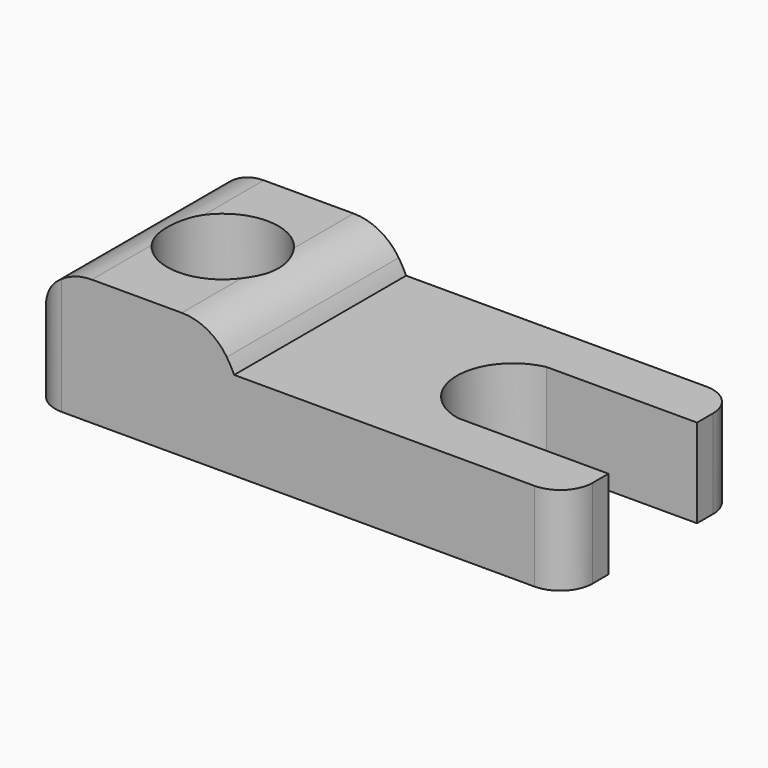
from build123d import *

# Parameters (mm, degrees)
F1_DEPTH     = 20
F2_R         = 1.6
F2_R_2       = 5.175
F3_DEPTH     = 7
F4_DEPTH     = 25
F5_R         = 3
F6_T1_DEPTH  = 28.6148731674
F7_DEPTH     = 25
F9_DEPTH     = 25
F10_T1_DEPTH = 35.1990481771


# Not quite as in the source:
# - a fillet or chamfer that OpenCascade refuses, or shapes differently, is made with other operations: its cross-section is extruded or revolved along the edge and cut away or added
# - a feature names something its author has since deleted; it is built from what else it names


with BuildPart() as f1:
    # F0 (on Front) → F1 (new body)
    with BuildSketch(Plane.XZ):
        with BuildLine():
            Line((-25, -4.125), (25, -4.125))
            Line((25, -4.125), (25, 4.125))
            Line((25, 4.125), (-5.9433734098, 4.125))
            ThreePointArc((-5.9433734098, 4.125), (-15, 9.8850100464), (-24.0566265902, 4.125))
            Line((-24.0566265902, 4.125), (-25, 4.125))
            Line((-25, 4.125), (-25, -4.125))
        make_face()
    extrude(amount=F1_DEPTH)

    # F2 (on face) → F3 (cut)
    with BuildSketch(Plane(origin=(0, 0, -4.125), x_dir=(1, 0, 0), z_dir=(0, 0, -1))):
        with Locations((-22.5875, 10)):
            Circle(F2_R)
        with Locations((-15, 10)):
            Circle(F2_R_2)
        with Locations((-15, 17.5875)):
            Circle(F2_R)
        with Locations((-15, 2.4125)):
            Circle(F2_R)
        with Locations((-7.4125, 10)):
            Circle(F2_R)
    extrude(amount=-F3_DEPTH, mode=Mode.SUBTRACT)

    # F4 (cut): a face of the model
    f4_faces = [f1.faces().sort_by_distance(p)[0] for p in [
        (-15, -10, 2.875),
    ]]
    extrude(f4_faces, amount=-F4_DEPTH, mode=Mode.SUBTRACT)

    # F5
    f5_edges = [f1.edges().sort_by_distance(p)[0] for p in [
        (25, 0, 0),
        (25, -20, 0),
        (-25, 0, 0),
        (-25, -20, 0),
    ]]
    fillet(f5_edges, radius=F5_R)

    # F6: fillet of radius 5 on 1 edges, made by hand

    # F6_s2 → F6_t1 (cut)
    with BuildSketch(Plane.XZ.offset(-4.3074365837)):
        with BuildLine():
            ThreePointArc((-24.0566265902, 4.125), (-24.7583155082, 2.7377445871), (-25, 1.2020253665))
            Line((-25, 1.2020253665), (-25, 4.125))
            Line((-25, 4.125), (-24.0566265902, 4.125))
        make_face()
    extrude(amount=F6_T1_DEPTH, mode=Mode.SUBTRACT)

    # F2 (on face) → F7 (cut)
    with BuildSketch(Plane(origin=(0, 0, -4.125), x_dir=(1, 0, 0), z_dir=(0, 0, -1))):
        with BuildLine():
            Line((25, 4.85), (25, 15.15))
            Line((25, 15.15), (11.0150124379, 15.15))
            ThreePointArc((11.0150124379, 15.15), (6.7728579207, 10), (11.0150124379, 4.85))
            Line((11.0150124379, 4.85), (25, 4.85))
        make_face()
    extrude(amount=-F7_DEPTH, mode=Mode.SUBTRACT)

    # F8 (on face) → F9 (cut)
    with BuildSketch(Plane.XZ.offset(20)):
        with BuildLine():
            Line((-21.3318682487, 7.625), (-8.6681317513, 7.625))
            ThreePointArc((-8.6681317513, 7.625), (-15, 9.8850100464), (-21.3318682487, 7.625))
        make_face()
    extrude(amount=-F9_DEPTH, mode=Mode.SUBTRACT)

    # F10: fillet of radius 5 on 2 edges, made by hand

    # F10_s2 → F10_t1 (cut)
    with BuildSketch(Plane.XZ.offset(-7.5995240885)):
        with BuildLine():
            ThreePointArc((-19.182398242, 7.625), (-21.55937639, 7.0238606347), (-23.3647964839, 5.3649899536))
            ThreePointArc((-23.3647964839, 5.3649899536), (-22.4347091347, 6.5726927603), (-21.3318682487, 7.625))
            Line((-21.3318682487, 7.625), (-19.182398242, 7.625))
        make_face()
        with BuildLine():
            ThreePointArc((-6.6352035161, 5.3649899536), (-8.44062361, 7.0238606347), (-10.817601758, 7.625))
            Line((-10.817601758, 7.625), (-8.6681317513, 7.625))
            ThreePointArc((-8.6681317513, 7.625), (-7.5652908653, 6.5726927603), (-6.6352035161, 5.3649899536))
        make_face()
    extrude(amount=F10_T1_DEPTH, mode=Mode.SUBTRACT)


solid = f1.part
